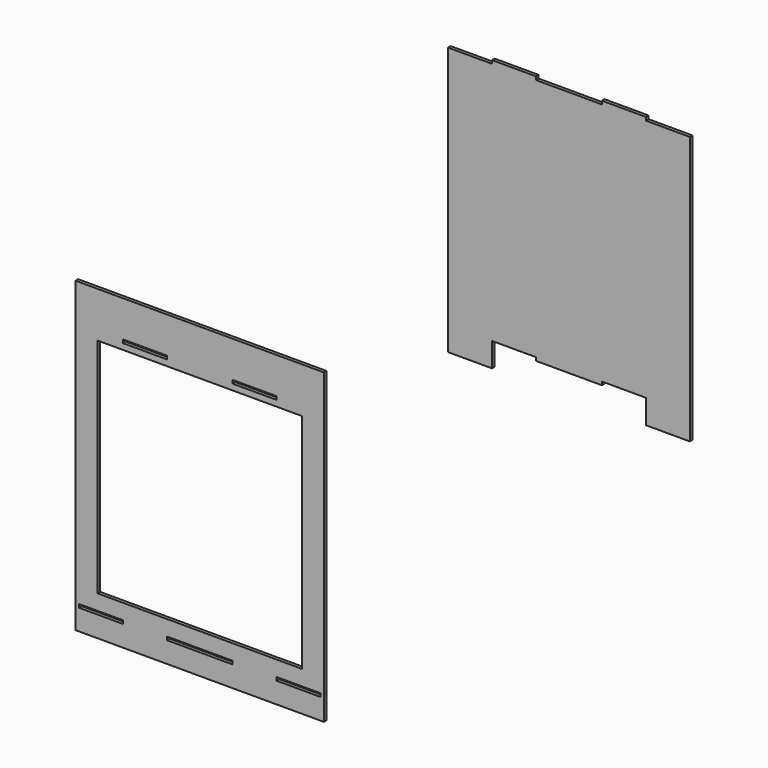
from build123d import *

# Parameters (mm, degrees)
F0_W     = 40
F0_H     = 19
F0_H_2   = 3
F0_W_2   = 186
F0_H_3   = 202.5581719875
F0_W_3   = 17
F0_H_4   = 14
F0_W_4   = 60
F1_DEPTH = 3
F3_DEPTH = 3


# Not quite as in the source:
# - a feature names something its author has since deleted; it is built from what else it names


with BuildPart() as f1:
    # F0 (on Front) → F1 (new body)
    with BuildSketch(Plane.XZ):
        with Locations((-90, -130.5)):
            Rectangle(F0_W, F0_H)
        with Locations((-50, 105.5)):
            Rectangle(F0_W, F0_H_2)
        with Locations((0, -2.7209140062)):
            Rectangle(F0_W_2, F0_H_3)
        Polygon((93, -104), (-93, -104), (-93, -118), (-70, -118), (-30, -118), (30, -118), (70, -118), (93, -118), align=None)
        Polygon((-70, 104), (-93, 104), (-93, 98.5581719875), (93, 98.5581719875), (93, 104), (70, 104), (30, 104), (-30, 104), align=None)
        with Locations((50, 105.5)):
            Rectangle(F0_W, F0_H_2)
        Polygon((-93, 104), (-110, 104), (-110, -104), (-93, -104), (-93, 98.5581719875), align=None)
        Polygon((110, -104), (110, 104), (93, 104), (93, 98.5581719875), (93, -104), align=None)
        with Locations((-101.5, -111)):
            Rectangle(F0_W_3, F0_H_4)
        Polygon((-93, -118), (-110, -118), (-110, -121), (-70, -121), (-70, -118), align=None)
        with Locations((0, -119.5)):
            Rectangle(F0_W_4, F0_H_2)
        with Locations((90, -130.5)):
            Rectangle(F0_W, F0_H)
        Polygon((110, -121), (110, -118), (93, -118), (70, -118), (70, -121), align=None)
        with Locations((101.5, -111)):
            Rectangle(F0_W_3, F0_H_4)
    extrude(amount=F1_DEPTH)


with BuildPart() as f1_1:
    # F2: moved
    add(f1.part.moved(Location((336, 0, 0))))


with BuildPart() as f3:
    # F0 (on Front) → F3 (new body)
    with BuildSketch(Plane.XZ):
        Polygon((-110, 104), (-110, 140), (-113, 140), (-113, -140), (-110, -140), (-110, -121), (-110, -118), (-110, -104), align=None)
        Polygon((110, 140), (-110, 140), (-110, 104), (-93, 104), (-70, 104), (-70, 107), (-30, 107), (-30, 104), (30, 104), (30, 107), (70, 107), (70, 104), (93, 104), (110, 104), align=None)
        Polygon((113, 140), (110, 140), (110, 104), (110, -104), (110, -118), (110, -121), (110, -140), (113, -140), align=None)
        Polygon((-70, -121), (-70, -140), (-30, -140), (-30, -121), (-30, -118), (-70, -118), align=None)
        Polygon((-93, 104), (-110, 104), (-110, -104), (-93, -104), (-93, 98.5581719875), align=None)
        with Locations((-101.5, -111)):
            Rectangle(F0_W_3, F0_H_4)
        with Locations((101.5, -111)):
            Rectangle(F0_W_3, F0_H_4)
        Polygon((110, -104), (110, 104), (93, 104), (93, 98.5581719875), (93, -104), align=None)
        with Locations((-90, -130.5)):
            Rectangle(F0_W, F0_H)
        with Locations((0, -130.5)):
            Rectangle(F0_W_4, F0_H)
        Polygon((30, -140), (70, -140), (70, -121), (70, -118), (30, -118), (30, -121), align=None)
        with Locations((90, -130.5)):
            Rectangle(F0_W, F0_H)
        Polygon((93, -104), (-93, -104), (-93, -118), (-70, -118), (-30, -118), (30, -118), (70, -118), (93, -118), align=None)
        Polygon((-70, 104), (-93, 104), (-93, 98.5581719875), (93, 98.5581719875), (93, 104), (70, 104), (30, 104), (-30, 104), align=None)
    extrude(amount=F3_DEPTH)


with BuildPart() as f3_1:
    # F4: moved
    add(f3.part.moved(Location((0, 0, -333))))


solid = Compound([f1_1.part, f3_1.part])
